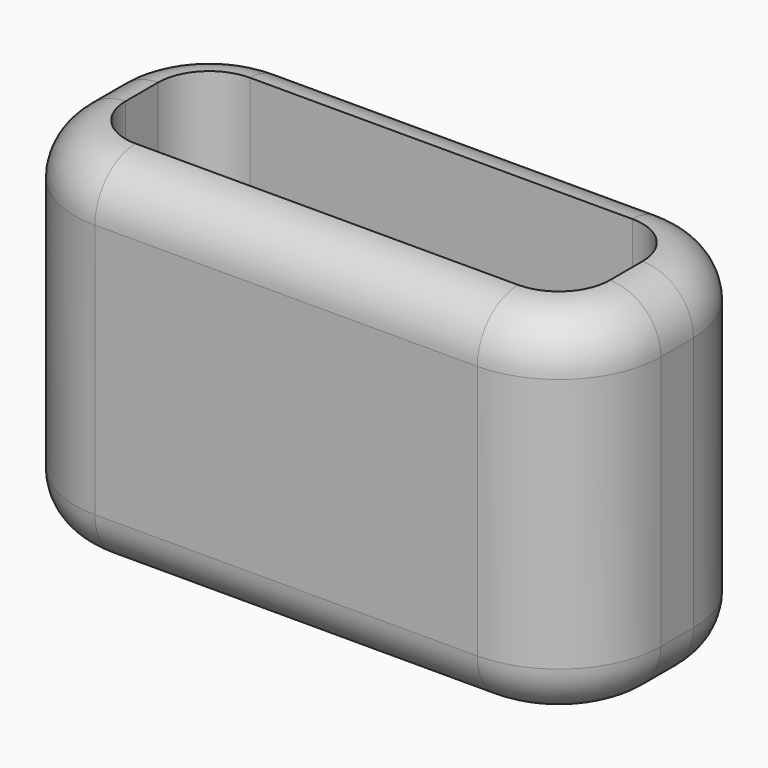
from build123d import *

# Parameters (mm, degrees)
F1_DEPTH = 7
F2_R     = 0.99999


# Not quite as in the source:
# - a fillet or chamfer is up to 0.001 mm smaller than in the source, because OpenCascade refuses the exact size


with BuildPart() as f1:
    # F0 (on Top) → F1 (new body)
    with BuildSketch(Plane.XY):
        with BuildLine():
            Line((-3.75, -2.4), (3.75, -2.4))
            ThreePointArc((3.75, -2.4), (5.1642135624, -1.8142135624), (5.75, -0.4))
            Line((5.75, -0.4), (5.75, 0.4))
            ThreePointArc((5.75, 0.4), (5.1642135624, 1.8142135624), (3.75, 2.4))
            Line((3.75, 2.4), (-3.75, 2.4))
            ThreePointArc((-3.75, 2.4), (-5.1642135624, 1.8142135624), (-5.75, 0.4))
            Line((-5.75, 0.4), (-5.75, -0.4))
            ThreePointArc((-5.75, -0.4), (-5.1642135624, -1.8142135624), (-3.75, -2.4))
        make_face()
        with BuildLine():
            ThreePointArc((4.75, -0.4), (4.4571067812, -1.1071067812), (3.75, -1.4))
            Line((3.75, -1.4), (-3.75, -1.4))
            ThreePointArc((-3.75, -1.4), (-4.4571067812, -1.1071067812), (-4.75, -0.4))
            Line((-4.75, -0.4), (-4.75, 0.4))
            ThreePointArc((-4.75, 0.4), (-4.4571067812, 1.1071067812), (-3.75, 1.4))
            Line((-3.75, 1.4), (3.75, 1.4))
            ThreePointArc((3.75, 1.4), (4.4571067812, 1.1071067812), (4.75, 0.4))
            Line((4.75, 0.4), (4.75, -0.4))
        make_face(mode=Mode.SUBTRACT)
    extrude(amount=F1_DEPTH)

    # F2 (radius 1 in the source; OpenCascade refuses exactly that, so slightly less here)
    f2_edges = [f1.edges().sort_by_distance(p)[0] for p in [
        (0, 2.4, 7),
        (0, 2.4, 0),
    ]]
    fillet(f2_edges, radius=F2_R)


solid = f1.part
